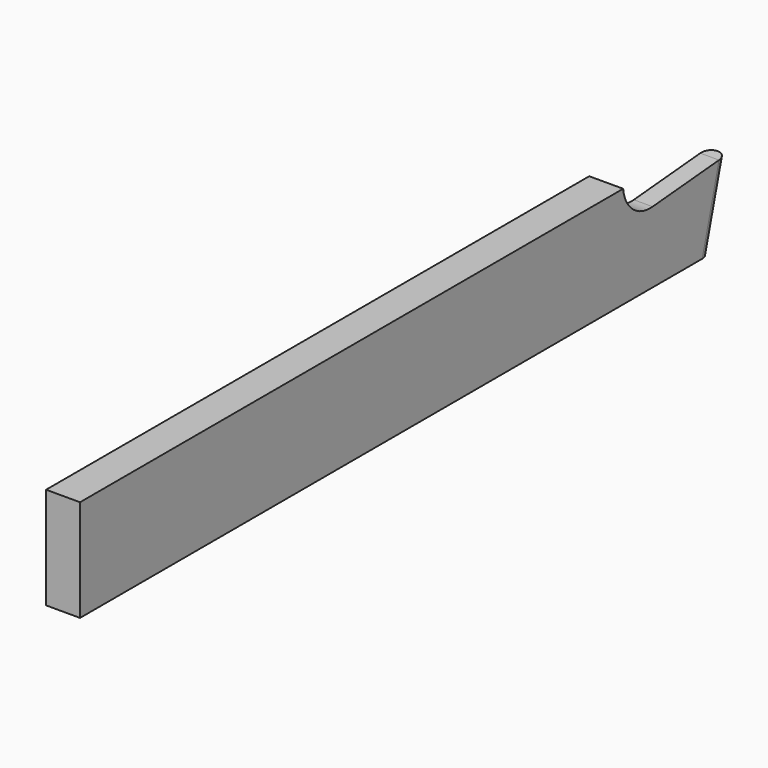
from build123d import *

# Parameters (mm, degrees)
F4_DEPTH     = 1.5875
F0_W         = 1.4224
F0_H         = 12.7
F5_DEPTH     = 25.4
F1_R         = 0.87629
F2_DEPTH     = 25.4
F7_T1_DEPTH  = 1.7526
F7_T6_DEPTH  = 12.9686376242
F7_T12_DEPTH = 12.9686376242
F7_T17_DEPTH = 10.3818412391


# Not quite as in the source:
# - a fillet or chamfer that OpenCascade refuses, or shapes differently, is made with other operations: its cross-section is extruded or revolved along the edge and cut away or added
# - a fillet or chamfer is up to 0.001 mm smaller than in the source, because OpenCascade refuses the exact size


with BuildPart() as f4:
    # F3 (on Right) → F4 (new body, symmetric)
    with BuildSketch(Plane.YZ):
        Polygon((35.5477839421, -4.7625), (38.1, 4.7625), (-38.1, 4.7625), (-38.1, -4.7625), align=None)
    extrude(amount=F4_DEPTH, both=True)

    # F0 (on face) → F5 (cut)
    with BuildSketch(Plane.XY.offset(4.7625)):
        with Locations((-0.8763, 31.75)):
            Rectangle(F0_W, F0_H)
    extrude(amount=-F5_DEPTH, mode=Mode.SUBTRACT)

    # F1 (radius 0.8763 in the source; OpenCascade refuses exactly that, so slightly less here)
    f1_edges = [f4.edges().sort_by_distance(p)[0] for p in [
        (1.5875, 36.823892, 0),
        (-0.1651, 36.823892, 0),
    ]]
    fillet(f1_edges, radius=F1_R)

    # F6 (on face) → F2 (cut)
    with BuildSketch(Plane.YZ.offset(1.5875)):
        Polygon((37.1927978359, 4.7625), (25.4, 4.7625), (25.4, 1.5875), (36.6047261297, 2.5677865143), align=None)
        Polygon((43.6932000767, 4.7625), (37.1927978359, 4.7625), (36.6047261297, 2.5677865143), (43.6932000767, 3.1879476263), align=None)
    extrude(amount=-F2_DEPTH, mode=Mode.SUBTRACT)

    # F7: fillet of radius 3.175 on 2 edges, made by hand

    # F7_s2 → F7_t1 (join)
    with BuildSketch(Plane.YZ.offset(-0.1651)):
        with BuildLine():
            ThreePointArc((25.4, 4.7625), (26.5256229175, 2.6151836003), (28.8385617484, 1.8883351718))
            Line((28.8385617484, 1.8883351718), (25.4, 1.5875))
            Line((25.4, 1.5875), (25.4, 4.7625))
        make_face()
    extrude(amount=F7_T1_DEPTH)


with BuildPart() as f7_tool4:
    # F7_s5 → F7_t6 (new body)
    with BuildSketch(Plane.XY.offset(8.2061376242)):
        with BuildLine():
            ThreePointArc((-0.1651, 28.0474550497), (-0.5432151257, 26.5447707848), (-1.5875, 25.4))
            Line((-1.5875, 25.4), (-0.1651, 25.4))
            Line((-0.1651, 25.4), (-0.1651, 28.0474550497))
        make_face()
    extrude(amount=-F7_T6_DEPTH)

    split(bisect_by=Plane(origin=(0, 0.0551082957, -0.6298907024), x_dir=(1, 0, 0), z_dir=(0, 0.0871557427, -0.9961946981)), keep=Keep.TOP)


with BuildPart() as f4_1:
    add(f4.part)

    # F7_t3: union F7_tool4
    add(f7_tool4.part)


with BuildPart() as f7_tool10:
    # F7_s11 → F7_t12 (new body)
    with BuildSketch(Plane.XY.offset(8.2061376242)):
        with BuildLine():
            ThreePointArc((-0.1651, 28.0474550497), (-0.5432151257, 26.5447707848), (-1.5875, 25.4))
            Line((-1.5875, 25.4), (-0.1651, 25.4))
            Line((-0.1651, 25.4), (-0.1651, 28.0474550497))
        make_face()
    extrude(amount=-F7_T12_DEPTH)

    split(bisect_by=Plane.XY.offset(4.7625), keep=Keep.BOTTOM)

    split(bisect_by=Plane(origin=(0, 0.0551082957, -0.6298907024), x_dir=(1, 0, 0), z_dir=(0, -0.0871557427, 0.9961946981)), keep=Keep.TOP)


with BuildPart() as f7_tool15:
    # F7_s16 → F7_t17 (new body)
    with BuildSketch(Plane.YZ.offset(1.5875)):
        with BuildLine():
            ThreePointArc((25.4, 4.7625), (26.5256229175, 2.6151836003), (28.8385617484, 1.8883351718))
            Line((28.8385617484, 1.8883351718), (25.4, 1.5875))
            Line((25.4, 1.5875), (25.4, 4.7625))
        make_face()
    extrude(amount=-F7_T17_DEPTH)

    split(bisect_by=Plane.YZ.offset(-0.1651), keep=Keep.BOTTOM)

    split(bisect_by=Plane.YZ.offset(-1.5875), keep=Keep.TOP)


with BuildPart() as f7_tool10_1:
    add(f7_tool10.part)

    # F7_t20: intersect F7_tool15
    add(f7_tool15.part, mode=Mode.INTERSECT)


with BuildPart() as f4_2:
    add(f4_1.part)

    # F7_t8: union F7_tool10
    add(f7_tool10_1.part)


solid = f4_2.part
